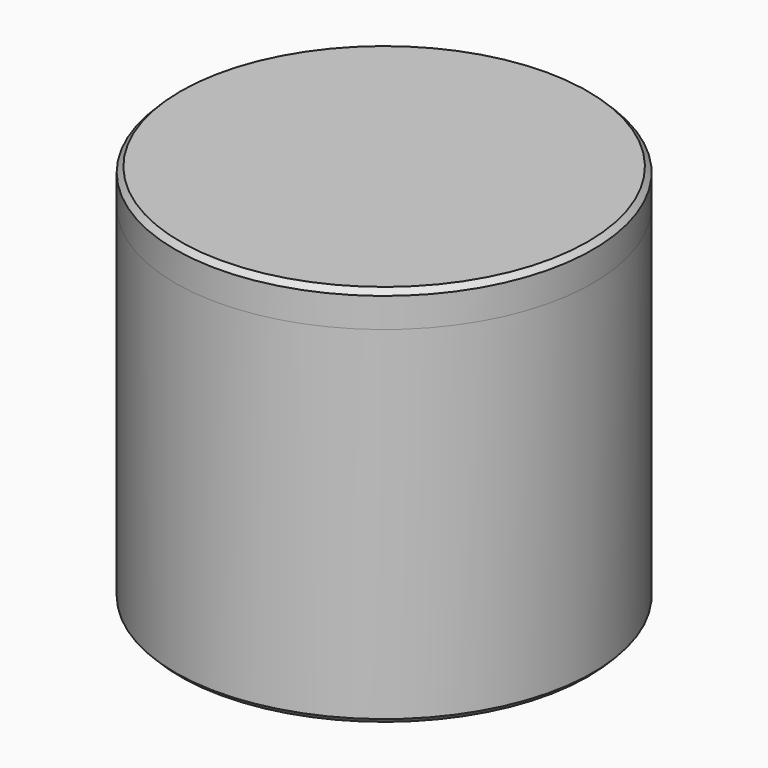
from build123d import *

# Parameters (mm, degrees)
F0_W    = 36.5
F0_H    = 10
F0_W_2  = 21
F0_H_2  = 21
F0_H_3  = 30
F0_W_3  = 3.25
F0_W_4  = 5
F4_SIZE = 1.5
F5_SIZE = 1.5
F6_SIZE = 3


# Not quite as in the source:
# - a feature names something its author has since deleted; it is built from what else it names


with BuildPart() as f1:
    # F0 (on Front) → F1 (revolve)
    with BuildSketch(Plane.XZ):
        Polygon((-60, 47.5), (-60, 37.5), (-44.75, 37.5), (-44.75, 47.5), (-50, 47.5), align=None)
        Polygon((-60, -47.5), (0, -47.5), (0, -32.5), (-25.75, -32.5), (-25.75, -9), (-41.5, -9), (-41.5, 32.5), (-41.5, 34.25), (-44.75, 37.5), (-60, 37.5), align=None)
        Polygon((-55, 52.5), (-60, 52.5), (-60, 47.5), (-50, 47.5), align=None)
    revolve(axis=Axis((0, 0, 13.6922076344), (0, 0, -1)))

    # F5
    f5_edges = [f1.edges().sort_by_distance(p)[0] for p in [
        (60, 0, -47.5),
    ]]
    chamfer(f5_edges, length=F5_SIZE)

    # F6
    f6_edges = [f1.edges().sort_by_distance(p)[0] for p in [
        (25.75, 0, -9),
    ]]
    chamfer(f6_edges, length=F6_SIZE)


with BuildPart() as f2:
    # F0 (on Front) → F2 (revolve)
    with BuildSketch(Plane.XZ):
        Polygon((0, 25.5), (0, 37.5), (-36.5, 37.5), (-36.5, 25.5), (-36.5, 4.5), (-21, 4.5), (-21, 25.5), align=None)
        with Locations((-18.25, 42.5)):
            Rectangle(F0_W, F0_H)
        with Locations((-10.5, 15)):
            Rectangle(F0_W_2, F0_H_2)
        with Locations((-10.5, -10.5)):
            Rectangle(F0_W_2, F0_H_3)
        Polygon((0, 47.5), (0, 62.5), (-60, 62.5), (-60, 52.5), (-55, 52.5), (-50, 47.5), (-44.75, 47.5), (-41.5, 47.5), (-36.5, 47.5), align=None)
    revolve(axis=Axis((0, 0, 13.6922076344), (0, 0, -1)))

    # F4
    f4_edges = [f2.edges().sort_by_distance(p)[0] for p in [
        (60, 0, 62.5),
    ]]
    chamfer(f4_edges, length=F4_SIZE)


with BuildPart() as f3:
    # F0 (on Front) → F3 (revolve)
    with BuildSketch(Plane.XZ):
        with Locations((-43.125, 42.5)):
            Rectangle(F0_W_3, F0_H)
        with Locations((-39, 42.5)):
            Rectangle(F0_W_4, F0_H)
        Polygon((-25.75, -32.5), (0, -32.5), (0, -25.5), (-21, -25.5), (-21, 4.5), (-36.5, 4.5), (-36.5, 25.5), (-36.5, 37.5), (-41.5, 37.5), (-41.5, 34.25), (-41.5, 32.5), (-41.5, -9), (-25.75, -9), align=None)
        Polygon((-41.5, 37.5), (-44.75, 37.5), (-41.5, 34.25), align=None)
    revolve(axis=Axis((0, 0, 13.6922076344), (0, 0, -1)))


solid = Compound([f1.part, f2.part, f3.part])
